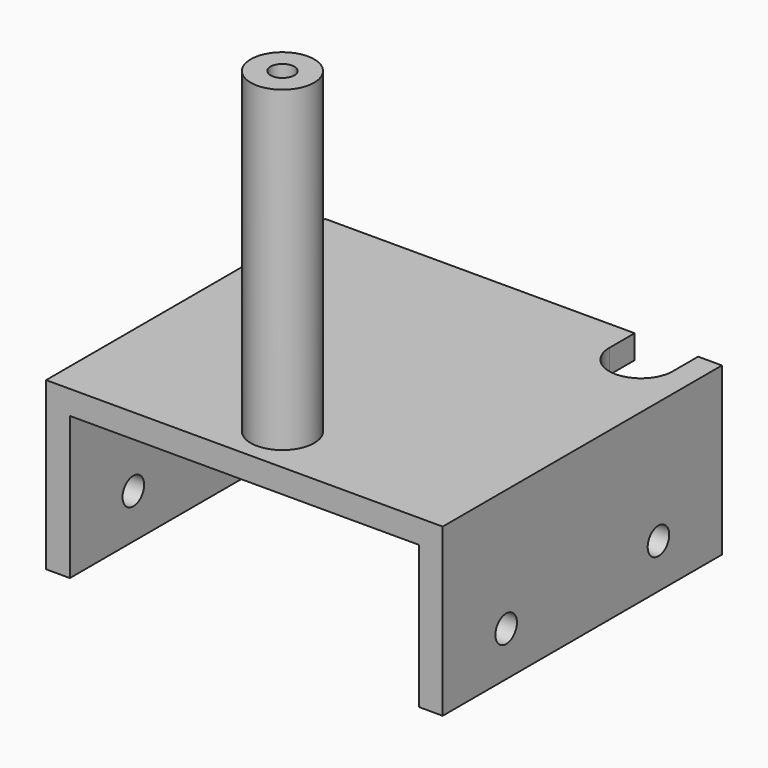
from build123d import *

# Parameters (mm, degrees)
F0_R     = 4
F0_W     = 3
F0_H     = 44
F0_R_2   = 1.5
F1_DEPTH = 3
F2_DEPTH = 18
F3_R     = 1.7
F4_DEPTH = 50
F5_DEPTH = 43


# Not quite as in the source:
# - a feature names something its author has since deleted; it is built from what else it names


with BuildPart() as f1:
    # F0 (on Top) → F1 (new body)
    with BuildSketch(Plane.XY):
        with BuildLine():
            Line((14, 22), (-22, 22))
            Line((-22, 22), (-22, -22))
            Line((-22, -22), (22, -22))
            Line((22, -22), (22, 18))
            ThreePointArc((22, 18), (18, 14), (14, 18))
            Line((14, 18), (14, 18.3849148452))
            Line((14, 18.3849148452), (14, 22))
        make_face()
        with Locations((0, -16)):
            Circle(F0_R, mode=Mode.SUBTRACT)
        with Locations((-23.5, 0)):
            Rectangle(F0_W, F0_H)
        Polygon((22, 18), (22, -22), (25, -22), (25, 22), (22, 22), align=None)
        with Locations((0, -16)):
            Circle(F0_R)
        with Locations((0, -16)):
            Circle(F0_R_2, mode=Mode.SUBTRACT)
    extrude(amount=F1_DEPTH)

    # F0 (on Top) → F2 (join)
    with BuildSketch(Plane.XY):
        with Locations((-23.5, 0)):
            Rectangle(F0_W, F0_H)
        Polygon((22, 18), (22, -22), (25, -22), (25, 22), (22, 22), align=None)
    extrude(amount=-F2_DEPTH)

    # F3 (on face) → F4 (cut, symmetric)
    with BuildSketch(Plane.YZ.offset(-22)):
        with Locations((-12, -12.4)):
            Circle(F3_R)
        with Locations((12, -12.4)):
            Circle(F3_R)
    extrude(amount=F4_DEPTH, both=True, mode=Mode.SUBTRACT)

    # F0 (on Top) → F5 (join)
    with BuildSketch(Plane.XY):
        with Locations((0, -16)):
            Circle(F0_R)
        with Locations((0, -16)):
            Circle(F0_R_2, mode=Mode.SUBTRACT)
    extrude(amount=F5_DEPTH)


solid = f1.part
